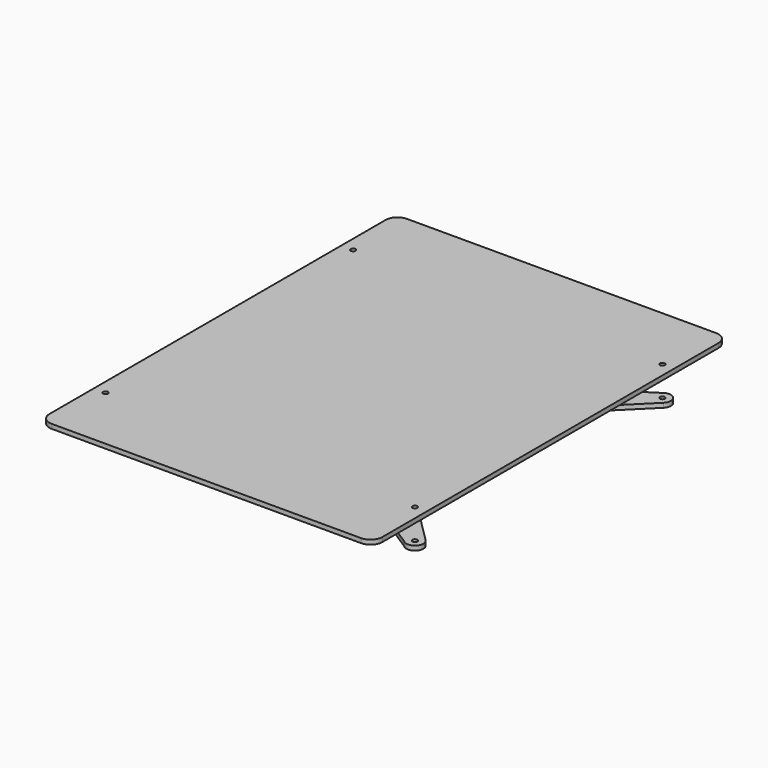
from build123d import *

# Parameters (mm, degrees)
F0_R     = 1.65
F0_R_2   = 3.555
F0_R_3   = 1.5
F0_W     = 10
F0_H     = 5
F0_R_4   = 2.55
F1_DEPTH = 3
F3_START = 20
F2_R     = 1.65
F3_DEPTH = 3


# Not quite as in the source:
# - a feature names something its author has since deleted; it is built from what else it names


with BuildPart() as f1:
    # F0 (on Top) → F1 (new body)
    with BuildSketch(Plane.XY):
        with BuildLine():
            Line((-17.3973424224, 55), (-100.4784052001, 108.5492745357))
            ThreePointArc((-100.4784052001, 108.5492745357), (-108.5492745357, 108.5215947999), (-108.5215947999, 100.4507254643))
            Line((-108.5215947999, 100.4507254643), (-35, 27.4317042255))
            Line((-35, 27.4317042255), (-35, -27.4317042255))
            Line((-35, -27.4317042255), (-108.5215947999, -100.4507254643))
            ThreePointArc((-108.5215947999, -100.4507254643), (-108.5492745357, -108.5215947999), (-100.4784052001, -108.5492745357))
            Line((-100.4784052001, -108.5492745357), (-17.3973424224, -55))
            Line((-17.3973424224, -55), (17.3973424224, -55))
            Line((17.3973424224, -55), (100.4784052001, -108.5492745357))
            ThreePointArc((100.4784052001, -108.5492745357), (108.5492745357, -108.5215947999), (108.5215947999, -100.4507254643))
            Line((108.5215947999, -100.4507254643), (35, -27.4317042255))
            Line((35, -27.4317042255), (35, 27.4317042255))
            Line((35, 27.4317042255), (108.5215947999, 100.4507254643))
            ThreePointArc((108.5215947999, 100.4507254643), (108.5492745357, 108.5215947999), (100.4784052001, 108.5492745357))
            Line((100.4784052001, 108.5492745357), (17.3973424224, 55))
            Line((17.3973424224, 55), (-17.3973424224, 55))
        make_face()
        with Locations((-104.5, -104.5)):
            Circle(F0_R, mode=Mode.SUBTRACT)
        with Locations((-20.8095, -44.445)):
            Circle(F0_R_2, mode=Mode.SUBTRACT)
        with Locations((-10, -10)):
            Circle(F0_R_3, mode=Mode.SUBTRACT)
        with Locations((104.5, -104.5)):
            Circle(F0_R, mode=Mode.SUBTRACT)
        with Locations((0, -49.5)):
            Rectangle(F0_W, F0_H, mode=Mode.SUBTRACT)
        with Locations((20.8095, -44.445)):
            Circle(F0_R_4, mode=Mode.SUBTRACT)
        Polygon((0, -40), (-20, -20), (20, -20), align=None, mode=Mode.SUBTRACT)
        with Locations((10, -10)):
            Circle(F0_R_3, mode=Mode.SUBTRACT)
        with Locations((-10, 10)):
            Circle(F0_R_3, mode=Mode.SUBTRACT)
        with Locations((-20.8095, 44.445)):
            Circle(F0_R_2, mode=Mode.SUBTRACT)
        with Locations((-104.5, 104.5)):
            Circle(F0_R, mode=Mode.SUBTRACT)
        with Locations((10, 10)):
            Circle(F0_R_3, mode=Mode.SUBTRACT)
        Polygon((-20, 20), (0, 40), (20, 20), align=None, mode=Mode.SUBTRACT)
        with Locations((0, 49.5)):
            Rectangle(F0_W, F0_H, mode=Mode.SUBTRACT)
        with Locations((20.8095, 44.445)):
            Circle(F0_R_4, mode=Mode.SUBTRACT)
        with Locations((104.5, 104.5)):
            Circle(F0_R, mode=Mode.SUBTRACT)
    extrude(amount=F1_DEPTH)


with BuildPart() as f3:
    # F2 (on Top) → F3 (new body)
    with BuildSketch(Plane.XY.offset(F3_START)):
        with BuildLine():
            Line((104.5, 150), (-104.5, 150))
            ThreePointArc((-104.5, 150), (-110.1568542495, 147.6568542495), (-112.5, 142))
            Line((-112.5, 142), (-112.5, -142))
            ThreePointArc((-112.5, -142), (-110.1568542495, -147.6568542495), (-104.5, -150))
            Line((-104.5, -150), (104.5, -150))
            ThreePointArc((104.5, -150), (110.1568542495, -147.6568542495), (112.5, -142))
            Line((112.5, -142), (112.5, 142))
            ThreePointArc((112.5, 142), (110.1568542495, 147.6568542495), (104.5, 150))
        make_face()
        with Locations((-104.5, -104.5)):
            Circle(F2_R, mode=Mode.SUBTRACT)
        with Locations((104.5, -104.5)):
            Circle(F2_R, mode=Mode.SUBTRACT)
        with Locations((-104.5, 104.5)):
            Circle(F2_R, mode=Mode.SUBTRACT)
        with Locations((104.5, 104.5)):
            Circle(F2_R, mode=Mode.SUBTRACT)
    extrude(amount=F3_DEPTH)


solid = Compound([f1.part, f3.part])
